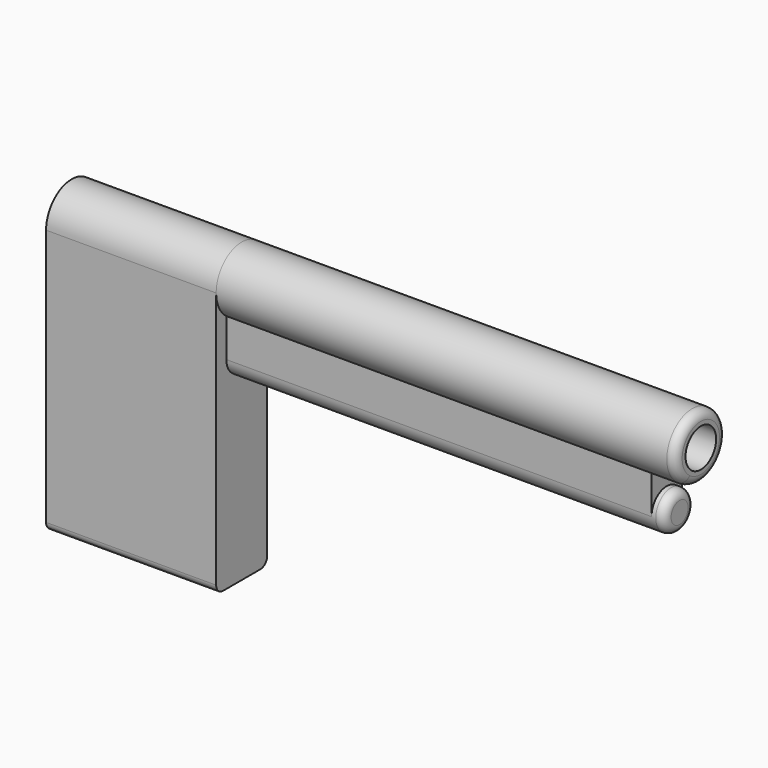
from build123d import *

# Parameters (mm, degrees)
F1_DEPTH = 103
F2_DEPTH = 100
F0_R     = 4.5
F3_DEPTH = 108
F4_R     = 2
F7_DEPTH = 40


# Not quite as in the source:
# - a fillet or chamfer that OpenCascade refuses, or shapes differently, is made with other operations: its cross-section is extruded or revolved along the edge and cut away or added
# - after a boolean that leaves OpenCascade's solid faulty, fix() repairs it


with BuildPart() as f1:
    # F0 (on Right) → F1 (new body)
    with BuildSketch(Plane.YZ):
        with BuildLine():
            ThreePointArc((4.5, -15), (0, -10.5), (-4.5, -15))
            ThreePointArc((-4.5, -15), (0, -19.5), (4.5, -15))
        make_face()
    extrude(amount=F1_DEPTH)

    # F0 (on Right) → F2 (join)
    with BuildSketch(Plane.YZ):
        with BuildLine():
            ThreePointArc((4.5, -6), (0, -7.5), (-4.5, -6))
            Line((-4.5, -6), (-4.5, -15))
            ThreePointArc((-4.5, -15), (0, -10.5), (4.5, -15))
            Line((4.5, -15), (4.5, -6))
        make_face()
    extrude(amount=F2_DEPTH)

    # F0 (on Right) → F3 (join)
    with BuildSketch(Plane.YZ):
        with BuildLine():
            ThreePointArc((4.5, -6), (6.7082039325, -3.3541019662), (7.5, 0))
            ThreePointArc((7.5, 0), (-3.3541019662, 6.7082039325), (-4.5, -6))
            ThreePointArc((-4.5, -6), (0, -7.5), (4.5, -6))
        make_face()
        Circle(F0_R, mode=Mode.SUBTRACT)
    extrude(amount=F3_DEPTH)

    # F4
    f4_edges = [f1.edges().sort_by_distance(p)[0] for p in [
        (108, 4.5, 6),
    ]]
    fillet(f4_edges, radius=F4_R)

    # F5: fillet of radius 2 on 1 edges, made by hand

    # F5_s1 → F5_t2 (revolve, cut)
    with BuildSketch(Plane.XY.offset(-15)):
        with BuildLine():
            ThreePointArc((101, 4.5), (102.4142135624, 3.9142135624), (103, 2.5))
            Line((103, 2.5), (103, 4.5))
            Line((103, 4.5), (101, 4.5))
        make_face()
    revolve(axis=Axis((103, 0, -15), (-1, 0, 0)), mode=Mode.SUBTRACT)

    # F6 (on Right) → F7 (join)
    with BuildSketch(Plane.YZ):
        with BuildLine():
            ThreePointArc((-7.5, -60.5), (-6.9142135624, -61.9142135624), (-5.5, -62.5))
            Line((-5.5, -62.5), (5.5, -62.5))
            ThreePointArc((5.5, -62.5), (6.9142135624, -61.9142135624), (7.5, -60.5))
            Line((7.5, -60.5), (7.5, 0))
            ThreePointArc((7.5, 0), (5.3033008589, 5.3033008589), (0, 7.5))
            ThreePointArc((0, 7.5), (-5.3033008589, 5.3033008589), (-7.5, 0))
            Line((-7.5, 0), (-7.5, -60.5))
        make_face()
    extrude(amount=-F7_DEPTH)

    add(f1.part.fix(), mode=Mode.REPLACE)


solid = f1.part
